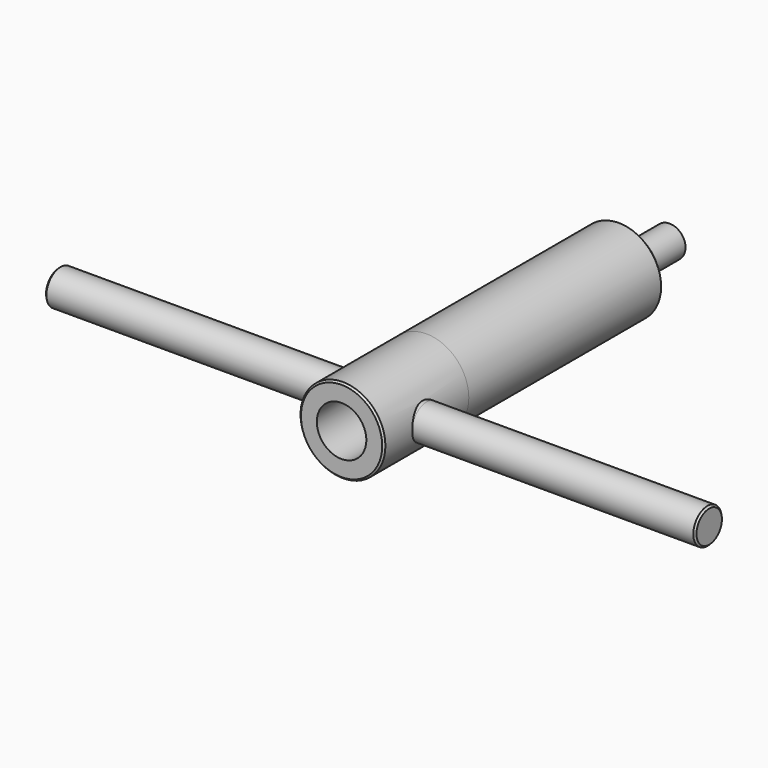
from build123d import *

# Parameters (mm, degrees)
F0_R           = 12
F1_DEPTH       = 30
F3_DEPTH       = 70
F2_R           = 2.5
F4_DEPTH       = 100.001
F6_D           = 14
F6_DEPTH       = 15
F6_TIP         = 4.2060243332
F8_R           = 5
F9_DEPTH       = 80
F9_DEPTH_BACK  = 3
F11_R          = 5
F12_DEPTH      = 80
F12_DEPTH_BACK = 3
F13_SIZE       = 0.5
F14_R          = 4.5
F15_DEPTH      = 16
F16_R          = 2.5
F17_DEPTH      = 116.001
F18_SIZE       = 2


with BuildPart() as f1:
    # F0 (on Front) → F1 (new body)
    with BuildSketch(Plane.XZ):
        Circle(F0_R)
    extrude(amount=F1_DEPTH)


with BuildPart() as f3:
    # F3 (new): a face of the model
    f3_faces = [f1.part.faces().sort_by_distance(p)[0] for p in [
        (0, 0, 0),
    ]]
    extrude(f3_faces, amount=F3_DEPTH)

    # F14 (on face) → F15 (join)
    with BuildSketch(Plane(origin=(0, 70, 0), x_dir=(-1, 0, 0), z_dir=(0, 1, 0))):
        Circle(F14_R)
    extrude(amount=F15_DEPTH)

    # F16 (on face) → F17 (cut, through all)
    with BuildSketch(Plane(origin=(0, 86, 0), x_dir=(-1, 0, 0), z_dir=(0, 1, 0))):
        Circle(F16_R)
    extrude(amount=-F17_DEPTH, mode=Mode.SUBTRACT)

    # F18
    f18_edges = [f3.edges().sort_by_distance(p)[0] for p in [
        (-12, 70, 0),
    ]]
    chamfer(f18_edges, length=F18_SIZE)


with BuildPart() as f1_1:
    add(f1.part)

    # F2 (on face) → F4 (cut, through all)
    with BuildSketch(Plane.XZ.offset(30)):
        Circle(F2_R)
    extrude(amount=-F4_DEPTH, mode=Mode.SUBTRACT)

    # F6
    with Locations(Plane.XZ.offset(30)):
        with Locations((0, 0)):
            Hole(F6_D / 2, depth=F6_DEPTH)
            with Locations((0, 0, -(F6_DEPTH + F6_TIP / 2))):  # 118° drill point
                Cone(0, F6_D / 2, F6_TIP, mode=Mode.SUBTRACT)

    # F8 (on offset) → F9 (join, two sides)
    with BuildSketch(Plane.YZ.offset(12)) as f9_sk:
        with Locations((-15, 0)):
            Circle(F8_R)
    extrude(amount=F9_DEPTH)
    extrude(f9_sk.sketch, amount=-F9_DEPTH_BACK)

    # F11 (on offset) → F12 (join, two sides)
    with BuildSketch(Plane.YZ.offset(-12)) as f12_sk:
        with Locations((-15, 0)):
            Circle(F11_R)
    extrude(amount=-F12_DEPTH)
    extrude(f12_sk.sketch, amount=F12_DEPTH_BACK)

    # F13
    f13_edges = [f1_1.edges().sort_by_distance(p)[0] for p in [
        (92, -20, 0),
        (-12, -30, 0),
        (-92, -20, 0),
    ]]
    chamfer(f13_edges, length=F13_SIZE)


solid = Compound([f3.part, f1_1.part])
